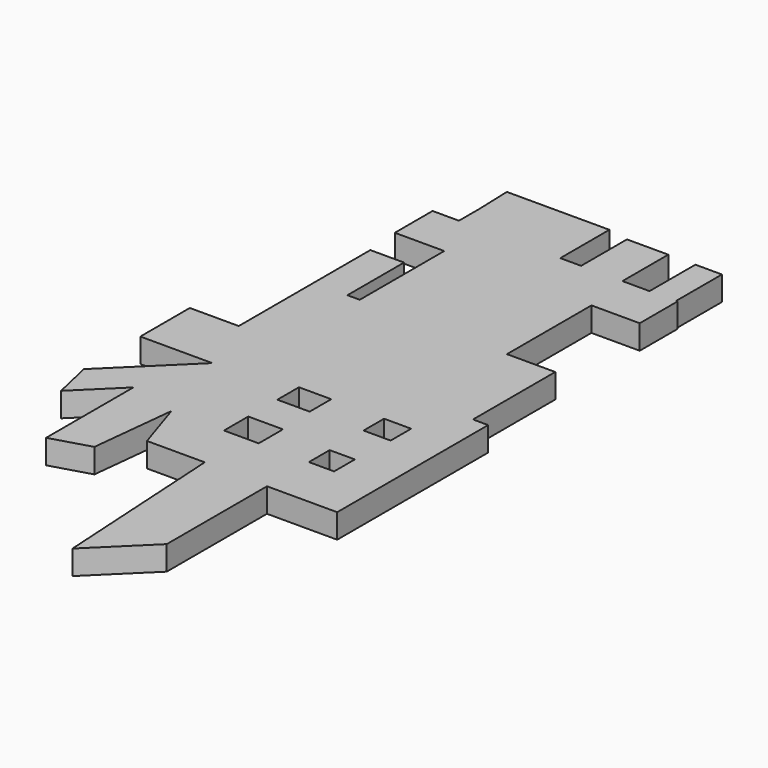
from build123d import *

# Parameters (mm, degrees)
F1_W     = 9.3304801267
F1_H     = 7.7842138708
F1_W_2   = 7.8273694962
F1_H_2   = 7.4135381728
F1_W_3   = 29.2622358538
F1_H_3   = 7.2785243392
F1_W_4   = 7.6639167964
F1_H_4   = 5.8850795031
F1_H_5   = 10.659635067
F2_DEPTH = 7


# Not quite as in the source:
# - a feature names something its author has since deleted; it is built from what else it names


with BuildPart() as f2:
    # F1 (on Top) → F2 (new body)
    with BuildSketch(Plane.XY):
        Polygon((-41.9203750789, 47.4954210222), (-41.9203750789, 16.0942748189), (-3.3160478342, 16.0942748189), (-3.3160478342, 27.0578376949), (-14.6702602506, 27.0578376949), (-14.6702602506, 34.84358266), (-3.3160478342, 34.84358266), (-3.3160478342, 47.4954210222), (-14.6702602506, 47.4954210222), (-14.6702602506, 57.5520098209), (0, 57.5520098209), (0, 16.0942748189), (27.8269369155, 16.0942748189), (27.8269369155, 18.2988718152), (27.8269369155, 27.0578376949), (13.8774756342, 27.0578376949), (13.8774756342, 57.5520098209), (27.8269369155, 57.5520098209), (27.8269369155, 71.1770653725), (27.4223256856, 71.1770653725), (19.7584088892, 71.1770653725), (11.9310393929, 71.1770653725), (11.9310393929, 87.7217799425), (0, 87.7217799425), (0, 71.1770653725), (-6.0202269815, 71.1770653725), (-35.2824628353, 71.1770653725), (-42.8935922682, 71.1770653725), (-42.8935922682, 57.5520098209), (-28.6197233945, 57.5520098209), (-28.6197233945, 27.0578376949), (-32.1881920099, 27.0578376949), (-32.1881920099, 47.4954210222), align=None)
        Polygon((-3.3160478342, 16.0942748189), (-41.9203750789, 16.0942748189), (-41.9203750789, 0), (-3.3160478342, 0), (-3.3160478342, 12.5654535368), align=None)
        Polygon((-3.3160478342, 27.0578376949), (-3.3160478342, 16.0942748189), (-3.3160478342, 12.5654535368), (11.9310393929, 12.5654535368), (11.9310393929, -2.6322980411), (27.8269369155, -2.6322980411), (27.8269369155, 16.0942748189), (0, 16.0942748189), (0, 57.5520098209), (-14.6702602506, 57.5520098209), (-14.6702602506, 47.4954210222), (-3.3160478342, 47.4954210222), (-3.3160478342, 34.84358266), (-14.6702602506, 34.84358266), (-14.6702602506, 27.0578376949), align=None)
        Polygon((-3.3160478342, 0), (-41.9203750789, 0), (-56.0475625098, 0), (-56.0475625098, -17.8618896753), (-35.2824628353, -17.8618896753), (-56.0475625098, -38.2491163909), (-53.4528233111, -49.7401021421), (-41.7488545561, -38.2491163909), (-41.7488545561, -69.7566494346), (-30.4708592594, -66.4205625653), (-27.8442800045, -41.9240482152), (-23.0254810303, -56.7511208355), (-6.3450210728, -56.7511208355), (-3.3160478342, -108.2752048969), (11.9310393929, -93.3055765817), (11.9310393929, -57.1217983961), (32.2053730488, -57.1217983961), (32.2053730488, -2.6322980411), (27.8269369155, -2.6322980411), (11.9310393929, -2.6322980411), (11.9310393929, 12.5654535368), (-3.3160478342, 12.5654535368), align=None)
        Polygon((-12.6465279609, -38.2491163909), (-12.6465279609, -34.5105081797), (-12.6465279609, -33.1628471613), (-2.621053718, -33.1628471613), (-2.621053718, -41.9242307544), (-12.6465279609, -41.9242307544), align=None, mode=Mode.SUBTRACT)
        with Locations((-7.9812878976, -18.7567416579)):
            Rectangle(F1_W, F1_H, mode=Mode.SUBTRACT)
        Polygon((11.9310393929, -41.9240482152), (11.9310393929, -38.2491163909), (11.9310393929, -34.5105081797), (19.2130599171, -34.5105081797), (19.2130599171, -41.9973358512), (11.9310393929, -41.9973358512), align=None, mode=Mode.SUBTRACT)
        with Locations((15.8447241411, -18.5714038089)):
            Rectangle(F1_W_2, F1_H_2, mode=Mode.SUBTRACT)
        with Locations((-20.6513449084, 74.8163275421)):
            Rectangle(F1_W_3, F1_H_3)
        Polygon((-35.6308221817, 88.9063850045), (-35.2824628353, 78.4555897117), (-6.0202269815, 78.4555897117), (-6.0202269815, 88.9063850045), align=None)
        with Locations((23.5903672874, 74.119605124)):
            Rectangle(F1_W_4, F1_H_4)
        with Locations((23.5903672874, 82.391962409)):
            Rectangle(F1_W_4, F1_H_5)
    extrude(amount=F2_DEPTH)


solid = f2.part
